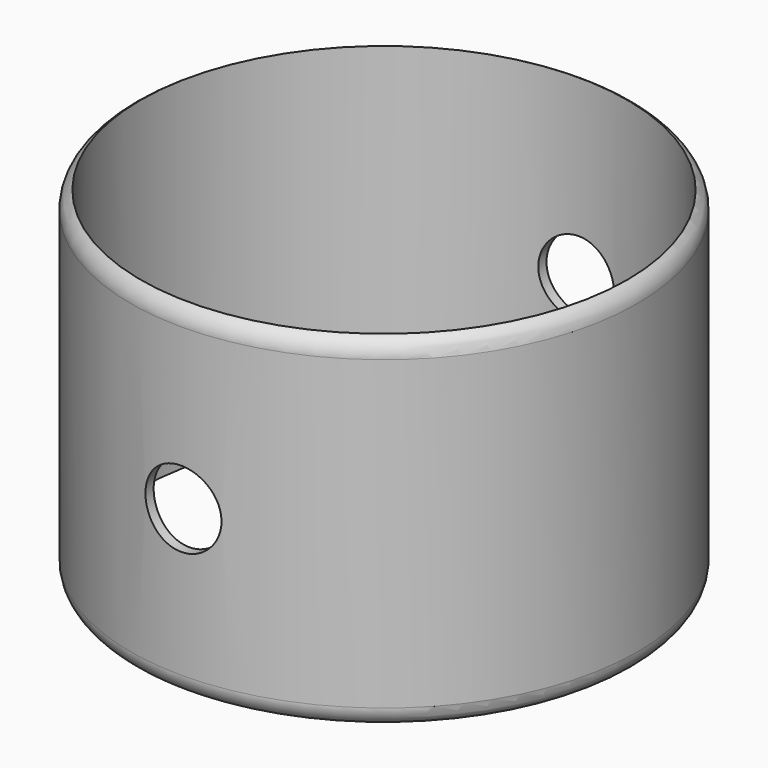
from build123d import *

# Parameters (mm, degrees)
F0_R     = 63.5
F1_DEPTH = 85.598
F2_T     = -2.54
F3_R     = 9.5217645964
F4_DEPTH = 92.964


# Not quite as in the source:
# - a fillet or chamfer that OpenCascade refuses, or shapes differently, is made with other operations: its cross-section is extruded or revolved along the edge and cut away or added


with BuildPart() as f1:
    # F0 (on Top) → F1 (new body)
    with BuildSketch(Plane.XY):
        Circle(F0_R)
    extrude(amount=F1_DEPTH)

    # F2
    f2_openings = [f1.faces().sort_by_distance(p)[0] for p in [
        (0, 0, 85.598),
        (0, 0, 0),
    ]]
    offset(amount=F2_T, openings=f2_openings)

    # F3 (on Front) → F4 (cut, symmetric)
    with BuildSketch(Plane.XZ):
        with Locations((0, 41.1053188145)):
            Circle(F3_R)
    extrude(amount=F4_DEPTH, both=True, mode=Mode.SUBTRACT)

    # F5: fillet of radius 5.08 on 2 edges, made by hand

    # F5_s1 → F5_t2 (revolve, cut)
    with BuildSketch(Plane.XZ):
        with BuildLine():
            ThreePointArc((63.5, 81.1985909488), (62.8194090512, 83.7385909488), (60.96, 85.598))
            Line((60.96, 85.598), (63.5, 85.598))
            Line((63.5, 85.598), (63.5, 81.1985909488))
        make_face()
    revolve(axis=Axis((0, 0, 85.598), (0, 0, 1)), mode=Mode.SUBTRACT)

    # F5_s3 → F5_t4 (revolve, cut)
    with BuildSketch(Plane.XZ):
        with BuildLine():
            ThreePointArc((63.5, 4.3994090512), (62.8194090512, 1.8594090512), (60.96, 0))
            Line((60.96, 0), (63.5, 0))
            Line((63.5, 0), (63.5, 4.3994090512))
        make_face()
    revolve(axis=Axis((0, 0, 0), (0, 0, 1)), mode=Mode.SUBTRACT)


solid = f1.part
